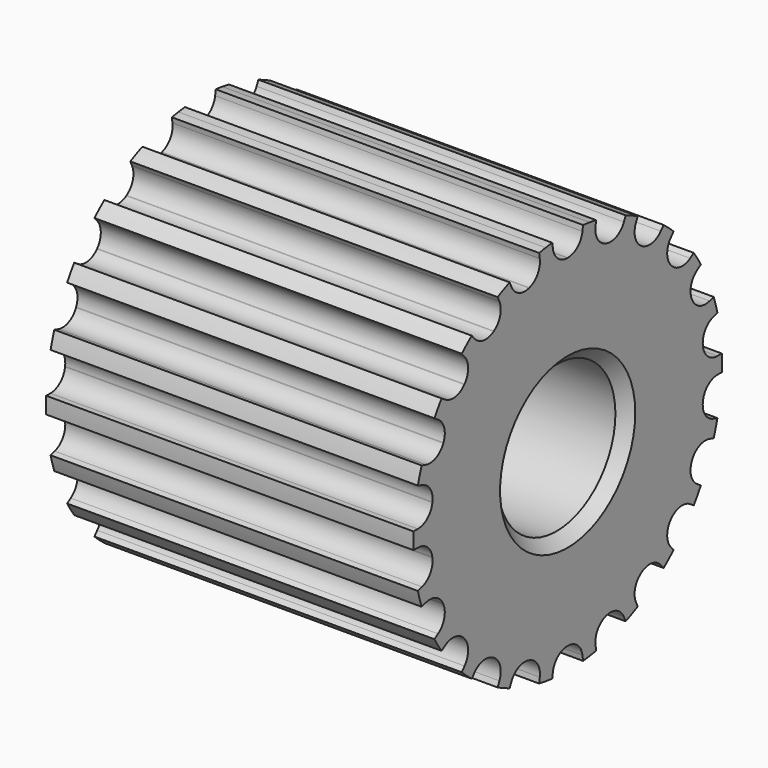
from build123d import *

# Parameters (mm, degrees)
F0_R     = 4
F1_DEPTH = 20
F2_SIZE  = 0.6


# Not quite as in the source:
# - a feature names something its author has since deleted; it is built from what else it names


with BuildPart() as f1:
    # F0 (on Right) → F1 (new body)
    with BuildSketch(Plane.YZ):
        with BuildLine():
            Line((-1.0058221805, 10.1576730476), (-1.0475098853, 10.4476180558))
            ThreePointArc((-1.0475098853, 10.4476180558), (-1.2711982189, 10.4227661918), (-1.4943025038, 10.3931256139))
            ThreePointArc((-1.4943025038, 10.3931256139), (-1.7167235223, 10.3587093959), (-1.9383557731, 10.3195337539))
            Line((-1.9383557731, 10.3195337539), (-1.8966678843, 10.0295887721))
            ThreePointArc((-1.8966678843, 10.0295887721), (-2.0456558496, 9.3459796694), (-2.6062476033, 8.927344142))
            ThreePointArc((-2.6062476033, 8.927344142), (-2.6201127786, 8.9232846546), (-2.633971631, 8.919203633))
            ThreePointArc((-2.633971631, 8.919203633), (-3.331902878, 8.9683034654), (-3.8268265142, 9.4628430628))
            Line((-3.8268265142, 9.4628430628), (-3.9485125225, 9.7292984773))
            ThreePointArc((-3.9485125225, 9.7292984773), (-4.3618576365, 9.5511359512), (-4.7671873745, 9.3554221998))
            Line((-4.7671873745, 9.3554221998), (-4.6455011971, 9.0889668625))
            ThreePointArc((-4.6455011971, 9.0889668625), (-4.5958591626, 8.3910739714), (-5.0157997538, 7.8314591763))
            ThreePointArc((-5.0157997538, 7.8314591763), (-5.0279596023, 7.8236578553), (-5.0401073171, 7.8158376539))
            ThreePointArc((-5.0401073171, 7.8158376539), (-5.723600466, 7.6663186434), (-6.3378041227, 8.0013898107))
            Line((-6.3378041227, 8.0013898107), (-6.5296301578, 8.2227689985))
            ThreePointArc((-6.5296301578, 8.2227689985), (-6.8760377064, 7.9353705307), (-7.2098098064, 7.6333899779))
            Line((-7.2098098064, 7.6333899779), (-7.0179836308, 7.4120109119))
            ThreePointArc((-7.0179836308, 7.4120109119), (-6.7737332988, 6.7563733639), (-7.0190016383, 6.1011159636))
            ThreePointArc((-7.0190016383, 6.1011159636), (-7.0284710415, 6.0902048257), (-7.0379234831, 6.0792789906))
            ThreePointArc((-7.0379234831, 6.0792789906), (-7.6516059839, 5.7432542782), (-8.3353305335, 5.8917115423))
            Line((-8.3353305335, 5.8917115423), (-8.581755991, 6.0500796781))
            ThreePointArc((-8.581755991, 6.0500796781), (-8.8331620947, 5.6767285833), (-9.0683363262, 5.2929458976))
            Line((-9.0683363262, 5.2929458976), (-8.8219107682, 5.1345779182))
            ThreePointArc((-8.8219107682, 5.1345779182), (-8.4028398482, 4.5743115681), (-8.4535657538, 3.8764966202))
            ThreePointArc((-8.4535657538, 3.8764966202), (-8.4595775568, 3.8633596209), (-8.4655689447, 3.8502132983))
            ThreePointArc((-8.4655689447, 3.8502132983), (-8.9597238908, 3.3549056078), (-9.6575780366, 3.3047218441))
            Line((-9.6575780366, 3.3047218441), (-9.9386389914, 3.3872488834))
            ThreePointArc((-9.9386389914, 3.3872488834), (-10.074676223, 2.9581918468), (-10.1922001683, 2.523698819))
            Line((-10.1922001683, 2.523698819), (-9.9111391611, 2.441171958))
            ThreePointArc((-9.9111391611, 2.441171958), (-9.3511982866, 2.0216662536), (-9.2032722471, 1.3378265751))
            ThreePointArc((-9.2032722471, 1.3378265751), (-9.2053394095, 1.3235279959), (-9.207384357, 1.3092262228))
            ThreePointArc((-9.207384357, 1.3092262228), (-9.5419782536, 0.6947624375), (-10.197426003, 0.450003236))
            Line((-10.197426003, 0.450003236), (-10.4903525681, 0.4500033289))
            ThreePointArc((-10.4903525681, 0.4500033289), (-10.5, 0), (-10.4903525681, -0.4500033289))
            Line((-10.4903525681, -0.4500033289), (-10.197426003, -0.450003236))
            ThreePointArc((-10.197426003, -0.450003236), (-9.5419782536, -0.6947624375), (-9.207384357, -1.3092262228))
            ThreePointArc((-9.207384357, -1.3092262228), (-9.2053394095, -1.3235279959), (-9.2032722471, -1.3378265751))
            ThreePointArc((-9.2032722471, -1.3378265751), (-9.3511982866, -2.0216662536), (-9.9111391611, -2.441171958))
            Line((-9.9111391611, -2.441171958), (-10.1922001683, -2.523698819))
            ThreePointArc((-10.1922001683, -2.523698819), (-10.074676223, -2.9581918468), (-9.9386389914, -3.3872488834))
            Line((-9.9386389914, -3.3872488834), (-9.6575780366, -3.3047218441))
            ThreePointArc((-9.6575780366, -3.3047218441), (-8.9597238908, -3.3549056078), (-8.4655689447, -3.8502132983))
            ThreePointArc((-8.4655689447, -3.8502132983), (-8.4595775568, -3.8633596209), (-8.4535657538, -3.8764966202))
            ThreePointArc((-8.4535657538, -3.8764966202), (-8.4028398482, -4.5743115681), (-8.8219107682, -5.1345779182))
            Line((-8.8219107682, -5.1345779182), (-9.0683363262, -5.2929458976))
            ThreePointArc((-9.0683363262, -5.2929458976), (-8.8331620947, -5.6767285833), (-8.581755991, -6.0500796781))
            Line((-8.581755991, -6.0500796781), (-8.3353305335, -5.8917115423))
            ThreePointArc((-8.3353305335, -5.8917115423), (-7.6516059839, -5.7432542782), (-7.0379234831, -6.0792789906))
            ThreePointArc((-7.0379234831, -6.0792789906), (-7.0284710415, -6.0902048257), (-7.0190016383, -6.1011159636))
            ThreePointArc((-7.0190016383, -6.1011159636), (-6.7737332988, -6.7563733639), (-7.0179836308, -7.4120109119))
            Line((-7.0179836308, -7.4120109119), (-7.2098098064, -7.6333899779))
            ThreePointArc((-7.2098098064, -7.6333899779), (-6.8760377064, -7.9353705307), (-6.5296301578, -8.2227689985))
            Line((-6.5296301578, -8.2227689985), (-6.3378041227, -8.0013898107))
            ThreePointArc((-6.3378041227, -8.0013898107), (-5.723600466, -7.6663186434), (-5.0401073171, -7.8158376539))
            ThreePointArc((-5.0401073171, -7.8158376539), (-5.0279596023, -7.8236578553), (-5.0157997538, -7.8314591763))
            ThreePointArc((-5.0157997538, -7.8314591763), (-4.5958591626, -8.3910739714), (-4.6455011971, -9.0889668625))
            Line((-4.6455011971, -9.0889668625), (-4.7671873745, -9.3554221998))
            ThreePointArc((-4.7671873745, -9.3554221998), (-4.3618576365, -9.5511359512), (-3.9485125225, -9.7292984773))
            Line((-3.9485125225, -9.7292984773), (-3.8268265142, -9.4628430628))
            ThreePointArc((-3.8268265142, -9.4628430628), (-3.331902878, -8.9683034654), (-2.633971631, -8.919203633))
            ThreePointArc((-2.633971631, -8.919203633), (-2.6201127786, -8.9232846546), (-2.6062476033, -8.927344142))
            ThreePointArc((-2.6062476033, -8.927344142), (-2.0456558496, -9.3459796694), (-1.8966678843, -10.0295887721))
            Line((-1.8966678843, -10.0295887721), (-1.9383557731, -10.3195337539))
            ThreePointArc((-1.9383557731, -10.3195337539), (-1.4943058019, -10.3931251397), (-1.0475098853, -10.4476180558))
            Line((-1.0475098853, -10.4476180558), (-1.0058221805, -10.1576730476))
            ThreePointArc((-1.0058221805, -10.1576730476), (-0.6702743343, -9.5437296773), (-0.0144472281, -9.2999887784))
            ThreePointArc((-0.0144472281, -9.2999887784), (0, -9.3), (0.0144472281, -9.2999887784))
            ThreePointArc((0.0144472281, -9.2999887784), (0.6702743343, -9.5437296773), (1.0058221805, -10.1576730476))
            Line((1.0058221805, -10.1576730476), (1.0475098853, -10.4476180558))
            ThreePointArc((1.0475098853, -10.4476180558), (1.4943058019, -10.3931251397), (1.9383557731, -10.3195337539))
            Line((1.9383557731, -10.3195337539), (1.8966678843, -10.0295887721))
            ThreePointArc((1.8966678843, -10.0295887721), (2.0456558496, -9.3459796694), (2.6062476033, -8.927344142))
            ThreePointArc((2.6062476033, -8.927344142), (2.6201127786, -8.9232846546), (2.633971631, -8.919203633))
            ThreePointArc((2.633971631, -8.919203633), (3.331902878, -8.9683034654), (3.8268265142, -9.4628430628))
            Line((3.8268265142, -9.4628430628), (3.9485125225, -9.7292984773))
            ThreePointArc((3.9485125225, -9.7292984773), (4.3618576365, -9.5511359512), (4.7671873745, -9.3554221998))
            Line((4.7671873745, -9.3554221998), (4.6455011971, -9.0889668625))
            ThreePointArc((4.6455011971, -9.0889668625), (4.5958591626, -8.3910739714), (5.0157997538, -7.8314591763))
            ThreePointArc((5.0157997538, -7.8314591763), (5.0279596023, -7.8236578553), (5.0401073171, -7.8158376539))
            ThreePointArc((5.0401073171, -7.8158376539), (5.723600466, -7.6663186434), (6.3378041227, -8.0013898107))
            Line((6.3378041227, -8.0013898107), (6.5296301578, -8.2227689985))
            ThreePointArc((6.5296301578, -8.2227689985), (6.8760377064, -7.9353705307), (7.2098098064, -7.6333899779))
            Line((7.2098098064, -7.6333899779), (7.0179836308, -7.4120109119))
            ThreePointArc((7.0179836308, -7.4120109119), (6.7737332988, -6.7563733639), (7.0190016383, -6.1011159636))
            ThreePointArc((7.0190016383, -6.1011159636), (7.0284710415, -6.0902048257), (7.0379234831, -6.0792789906))
            ThreePointArc((7.0379234831, -6.0792789906), (7.6516059839, -5.7432542782), (8.3353305335, -5.8917115423))
            Line((8.3353305335, -5.8917115423), (8.581755991, -6.0500796781))
            ThreePointArc((8.581755991, -6.0500796781), (8.8331620947, -5.6767285833), (9.0683363262, -5.2929458976))
            Line((9.0683363262, -5.2929458976), (8.8219107682, -5.1345779182))
            ThreePointArc((8.8219107682, -5.1345779182), (8.4028398482, -4.5743115681), (8.4535657538, -3.8764966202))
            ThreePointArc((8.4535657538, -3.8764966202), (8.4595775568, -3.8633596209), (8.4655689447, -3.8502132983))
            ThreePointArc((8.4655689447, -3.8502132983), (8.9597238908, -3.3549056078), (9.6575780366, -3.3047218441))
            Line((9.6575780366, -3.3047218441), (9.9386389914, -3.3872488834))
            ThreePointArc((9.9386389914, -3.3872488834), (10.074676223, -2.9581918468), (10.1922001683, -2.523698819))
            Line((10.1922001683, -2.523698819), (9.9111391611, -2.441171958))
            ThreePointArc((9.9111391611, -2.441171958), (9.3511982866, -2.0216662536), (9.2032722471, -1.3378265751))
            ThreePointArc((9.2032722471, -1.3378265751), (9.2053394095, -1.3235279959), (9.207384357, -1.3092262228))
            ThreePointArc((9.207384357, -1.3092262228), (9.5419782536, -0.6947624375), (10.197426003, -0.450003236))
            Line((10.197426003, -0.450003236), (10.4903525681, -0.4500033289))
            ThreePointArc((10.4903525681, -0.4500033289), (10.5, 0), (10.4903525681, 0.4500033289))
            Line((10.4903525681, 0.4500033289), (10.197426003, 0.450003236))
            ThreePointArc((10.197426003, 0.450003236), (9.5419782536, 0.6947624375), (9.207384357, 1.3092262228))
            ThreePointArc((9.207384357, 1.3092262228), (9.2053394095, 1.3235279959), (9.2032722471, 1.3378265751))
            ThreePointArc((9.2032722471, 1.3378265751), (9.3511982866, 2.0216662536), (9.9111391611, 2.441171958))
            Line((9.9111391611, 2.441171958), (10.1922001683, 2.523698819))
            ThreePointArc((10.1922001683, 2.523698819), (10.074676223, 2.9581918468), (9.9386389914, 3.3872488834))
            Line((9.9386389914, 3.3872488834), (9.6575780366, 3.3047218441))
            ThreePointArc((9.6575780366, 3.3047218441), (8.9597238908, 3.3549056078), (8.4655689447, 3.8502132983))
            ThreePointArc((8.4655689447, 3.8502132983), (8.4595775568, 3.8633596209), (8.4535657538, 3.8764966202))
            ThreePointArc((8.4535657538, 3.8764966202), (8.4028398482, 4.5743115681), (8.8219107682, 5.1345779182))
            Line((8.8219107682, 5.1345779182), (9.0683363262, 5.2929458976))
            ThreePointArc((9.0683363262, 5.2929458976), (8.8331620947, 5.6767285833), (8.581755991, 6.0500796781))
            Line((8.581755991, 6.0500796781), (8.3353305335, 5.8917115423))
            ThreePointArc((8.3353305335, 5.8917115423), (7.6516059839, 5.7432542782), (7.0379234831, 6.0792789906))
            ThreePointArc((7.0379234831, 6.0792789906), (7.0284710415, 6.0902048257), (7.0190016383, 6.1011159636))
            ThreePointArc((7.0190016383, 6.1011159636), (6.7737332988, 6.7563733639), (7.0179836308, 7.4120109119))
            Line((7.0179836308, 7.4120109119), (7.2098098064, 7.6333899779))
            ThreePointArc((7.2098098064, 7.6333899779), (6.8760377064, 7.9353705307), (6.5296301578, 8.2227689985))
            Line((6.5296301578, 8.2227689985), (6.3378041227, 8.0013898107))
            ThreePointArc((6.3378041227, 8.0013898107), (5.723600466, 7.6663186434), (5.0401073171, 7.8158376539))
            ThreePointArc((5.0401073171, 7.8158376539), (5.0279596023, 7.8236578553), (5.0157997538, 7.8314591763))
            ThreePointArc((5.0157997538, 7.8314591763), (4.5958591626, 8.3910739714), (4.6455011971, 9.0889668625))
            Line((4.6455011971, 9.0889668625), (4.7671873745, 9.3554221998))
            ThreePointArc((4.7671873745, 9.3554221998), (4.3618576365, 9.5511359512), (3.9485125225, 9.7292984773))
            Line((3.9485125225, 9.7292984773), (3.8268265142, 9.4628430628))
            ThreePointArc((3.8268265142, 9.4628430628), (3.331902878, 8.9683034654), (2.633971631, 8.919203633))
            ThreePointArc((2.633971631, 8.919203633), (2.6201127786, 8.9232846546), (2.6062476033, 8.927344142))
            ThreePointArc((2.6062476033, 8.927344142), (2.0456558496, 9.3459796694), (1.8966678843, 10.0295887721))
            Line((1.8966678843, 10.0295887721), (1.9383557731, 10.3195337539))
            ThreePointArc((1.9383557731, 10.3195337539), (1.7167235223, 10.3587093959), (1.4943025038, 10.3931256139))
            ThreePointArc((1.4943025038, 10.3931256139), (1.2711982189, 10.4227661918), (1.0475098853, 10.4476180558))
            Line((1.0475098853, 10.4476180558), (1.0058221805, 10.1576730476))
            ThreePointArc((1.0058221805, 10.1576730476), (0.6702743343, 9.5437296773), (0.0144472281, 9.2999887784))
            ThreePointArc((0.0144472281, 9.2999887784), (0, 9.3), (-0.0144472281, 9.2999887784))
            ThreePointArc((-0.0144472281, 9.2999887784), (-0.6702743343, 9.5437296773), (-1.0058221805, 10.1576730476))
        make_face()
        Circle(F0_R, mode=Mode.SUBTRACT)
    extrude(amount=F1_DEPTH)

    # F2
    f2_edges = [f1.edges().sort_by_distance(p)[0] for p in [
        (20, -4, 0),
        (0, -4, 0),
    ]]
    chamfer(f2_edges, length=F2_SIZE)


solid = f1.part
